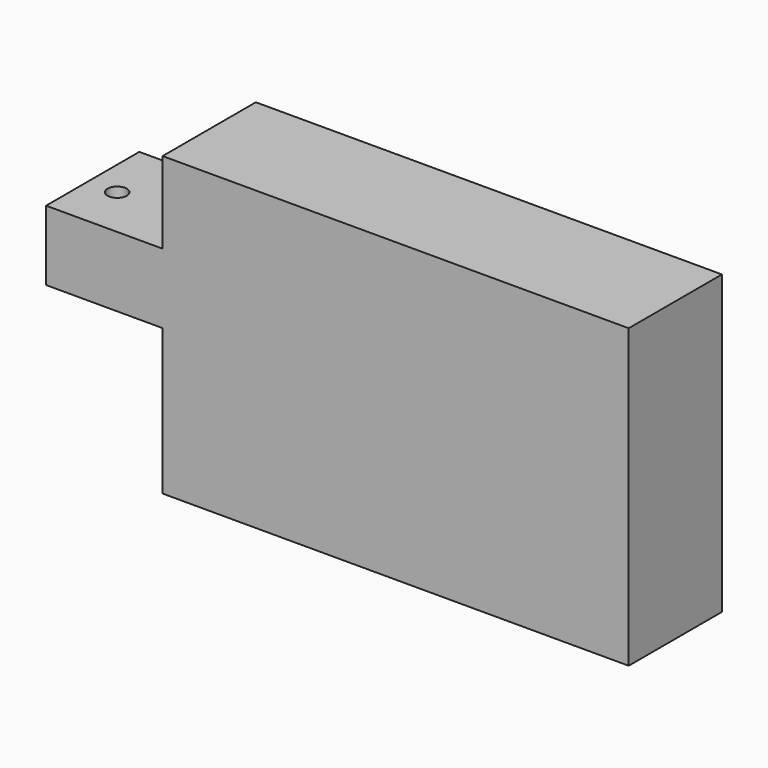
from build123d import *

# Parameters (mm, degrees)
F0_W     = 100
F0_H     = 20
F1_DEPTH = 51
F2_W     = 20
F2_H     = 20
F3_DEPTH = 14
F5_D     = 3.3
F5_DEPTH = 7
F5_TIP   = 0.9914200214
F6_W     = 20
F6_H     = 20
F7_DEPTH = 25


with BuildPart() as f1:
    # F0 (on Top) → F1 (new body)
    with BuildSketch(Plane.XY):
        with Locations((50, 10)):
            Rectangle(F0_W, F0_H)
    extrude(amount=F1_DEPTH)

    # F2 (on face) → F3 (cut)
    with BuildSketch(Plane.XY.offset(51)):
        with Locations((10, 10)):
            Rectangle(F2_W, F2_H)
    extrude(amount=-F3_DEPTH, mode=Mode.SUBTRACT)

    # F5
    with Locations(Plane.XY.offset(37)):
        with Locations((5, 9), (15, 9)):
            Hole(F5_D / 2, depth=F5_DEPTH)
            with Locations((0, 0, -(F5_DEPTH + F5_TIP / 2))):  # 118° drill point
                Cone(0, F5_D / 2, F5_TIP, mode=Mode.SUBTRACT)

    # F6 (on face) → F7 (cut)
    with BuildSketch(Plane(origin=(0, 0, 0), x_dir=(1, 0, 0), z_dir=(0, 0, -1))):
        with Locations((10, -10)):
            Rectangle(F6_W, F6_H)
    extrude(amount=-F7_DEPTH, mode=Mode.SUBTRACT)


solid = f1.part
